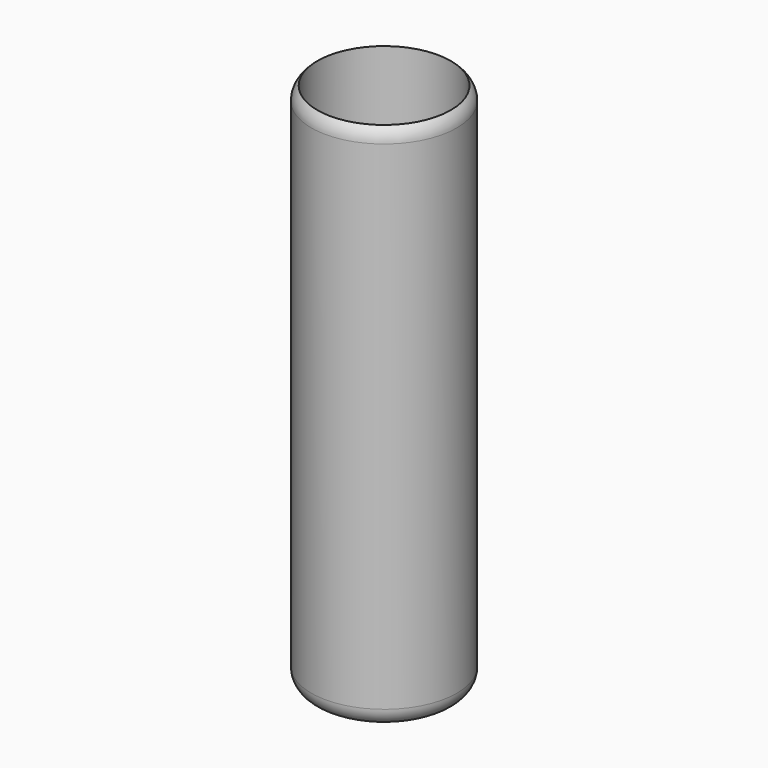
from build123d import *

# Parameters (mm, degrees)
F0_R     = 30.3497039052
F1_DEPTH = 220.726
F2_T     = -2.54


# Not quite as in the source:
# - a fillet or chamfer that OpenCascade refuses, or shapes differently, is made with other operations: its cross-section is extruded or revolved along the edge and cut away or added


with BuildPart() as f1:
    # F0 (on Top) → F1 (new body)
    with BuildSketch(Plane.XY):
        Circle(F0_R)
    extrude(amount=F1_DEPTH)

    # F2
    f2_openings = [f1.faces().sort_by_distance(p)[0] for p in [
        (0, 0, 220.726),
    ]]
    offset(amount=F2_T, openings=f2_openings)

    # F3: fillet of radius 7.62 on 3 edges, made by hand

    # F3_s1 → F3_t2 (revolve, cut)
    with BuildSketch(Plane.XZ):
        with BuildLine():
            ThreePointArc((30.3497039052, 7.62), (28.1178575778, 2.2318463274), (22.7297039052, 0))
            Line((22.7297039052, 0), (30.3497039052, 0))
            Line((30.3497039052, 0), (30.3497039052, 7.62))
        make_face()
    revolve(axis=Axis((0, 0, 0), (0, 0, 1)), mode=Mode.SUBTRACT)

    # F3_s3 → F3_t4 (revolve, cut)
    with BuildSketch(Plane.XZ):
        with BuildLine():
            ThreePointArc((30.3497039052, 215.0463873372), (29.6857803855, 218.1572393105), (27.8097039052, 220.726))
            Line((27.8097039052, 220.726), (30.3497039052, 220.726))
            Line((30.3497039052, 220.726), (30.3497039052, 215.0463873372))
        make_face()
    revolve(axis=Axis((0, 0, 220.726), (0, 0, 1)), mode=Mode.SUBTRACT)


solid = f1.part
